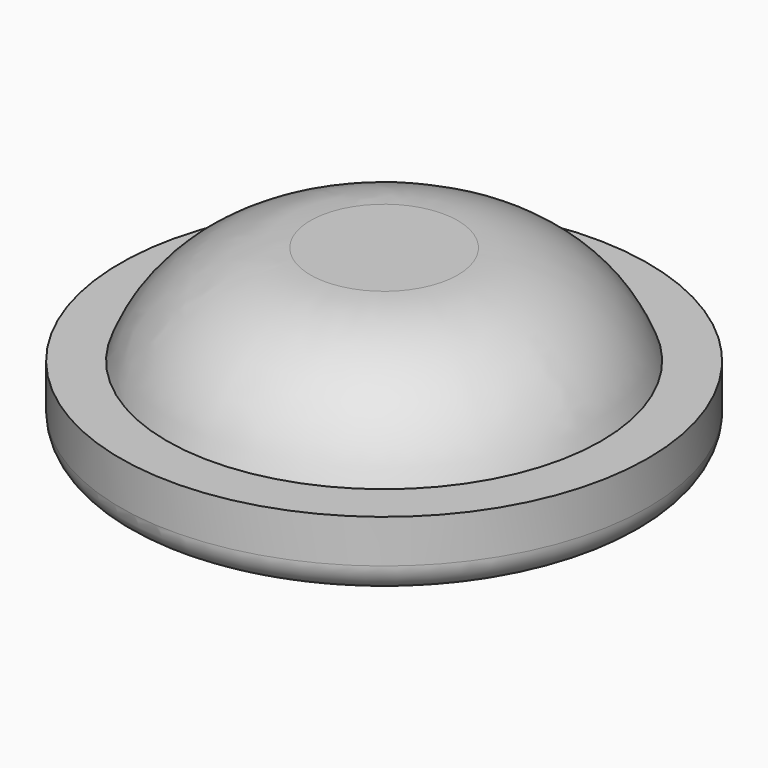
from build123d import *

# Parameters (mm, degrees)
F0_R     = 38.2508515855
F1_DEPTH = 17.526
F3_R     = 46.4966196034
F4_DEPTH = 12.7
F5_R     = 5.08
F6_W     = 8.4483027458
F6_H     = 6.8974085152
F8_DEPTH = 9.652
F7_W     = 9.7811389714
F7_H     = 6.7780073732
F9_DEPTH = 10.668


# Not quite as in the source:
# - a fillet or chamfer that OpenCascade refuses, or shapes differently, is made with other operations: its cross-section is extruded or revolved along the edge and cut away or added


with BuildPart() as f1:
    # F0 (on Top) → F1 (new body)
    with BuildSketch(Plane.XY):
        Circle(F0_R)
    extrude(amount=F1_DEPTH)

    # F2: fillet of radius 26.9812507731 on 1 edges, made by hand

    # F2_s1 → F2_t2 (revolve, cut)
    with BuildSketch(Plane.XZ):
        with BuildLine():
            ThreePointArc((38.2508515855, 0), (28.3570882092, 12.7157030349), (12.9805898912, 17.526))
            Line((12.9805898912, 17.526), (38.2508515855, 17.526))
            Line((38.2508515855, 17.526), (38.2508515855, 0))
        make_face()
    revolve(axis=Axis((0, 0, 17.526), (0, 0, 1)), mode=Mode.SUBTRACT)

    # F3 (on face) → F4 (join)
    with BuildSketch(Plane(origin=(0, 0, 0), x_dir=(1, 0, 0), z_dir=(0, 0, -1))):
        Circle(F3_R)
    extrude(amount=F4_DEPTH)

    # F5
    f5_edges = [f1.edges().sort_by_distance(p)[0] for p in [
        (-46.49662, 0, -12.7),
    ]]
    fillet(f5_edges, radius=F5_R)

    # F6 (on face) → F8 (join)
    with BuildSketch(Plane(origin=(0, 0, -12.7), x_dir=(1, 0, 0), z_dir=(0, 0, -1))):
        with Locations((-15.9282591194, 18.548514694)):
            Rectangle(F6_W, F6_H)
    extrude(amount=F8_DEPTH)

    # F7 (on face) → F9 (join)
    with BuildSketch(Plane(origin=(0, 0, -12.7), x_dir=(1, 0, 0), z_dir=(0, 0, -1))):
        with Locations((20.9769504145, -18.5471354052)):
            Rectangle(F7_W, F7_H)
    extrude(amount=F9_DEPTH)


solid = f1.part
